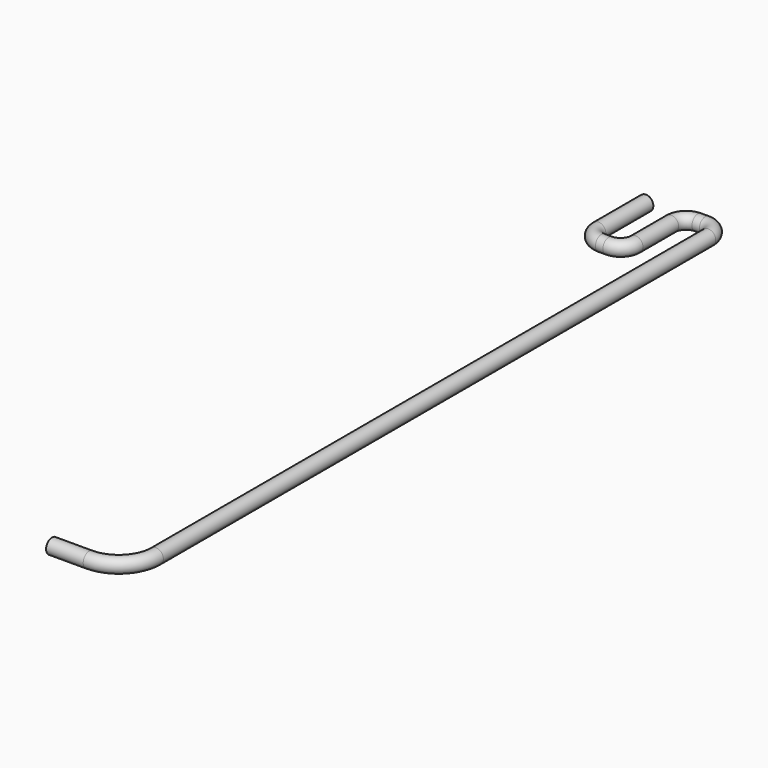
from build123d import *

# Parameters (mm, degrees)
F2_R = 1


# Not quite as in the source:
# - a feature names something its author has since deleted; it is built from what else it names


with BuildPart() as f3:
    # F3: sweep along a path in F0
    with BuildLine(Plane.XY) as f3_path:
        Line((-73.4692310878, 100), (-73.4692310878, 92))
        ThreePointArc((-73.4692310878, 92), (-72.8834446502, 90.5857864376), (-71.4692310878, 90))
        Line((-71.4692310878, 90), (-70.4692310878, 90))
        ThreePointArc((-70.4692310878, 90), (-69.0550175254, 90.5857864376), (-68.4692310878, 92))
        Line((-68.4692310878, 92), (-68.4692310878, 98))
        ThreePointArc((-68.4692310878, 98), (-67.8834446502, 99.4142135624), (-66.4692310878, 100))
        Line((-66.4692310878, 100), (-65.4692310878, 100))
        ThreePointArc((-65.4692310878, 100), (-64.0550175254, 99.4142135624), (-63.4692310878, 98))
        Line((-63.4692310878, 98), (-63.4692310878, 5))
        ThreePointArc((-63.4692310878, 5), (-64.9336971819, 1.4644660941), (-68.4692310878, 0))
        Line((-68.4692310878, 0), (-73.4692310878, 0))
    # F2 (on plane+point) → F3 (sweep)
    with BuildSketch(Plane.XZ.offset(-100)):
        with Locations((-73.4692310878, 0)):
            Circle(F2_R)
    sweep(path=f3_path.line)


solid = f3.part
